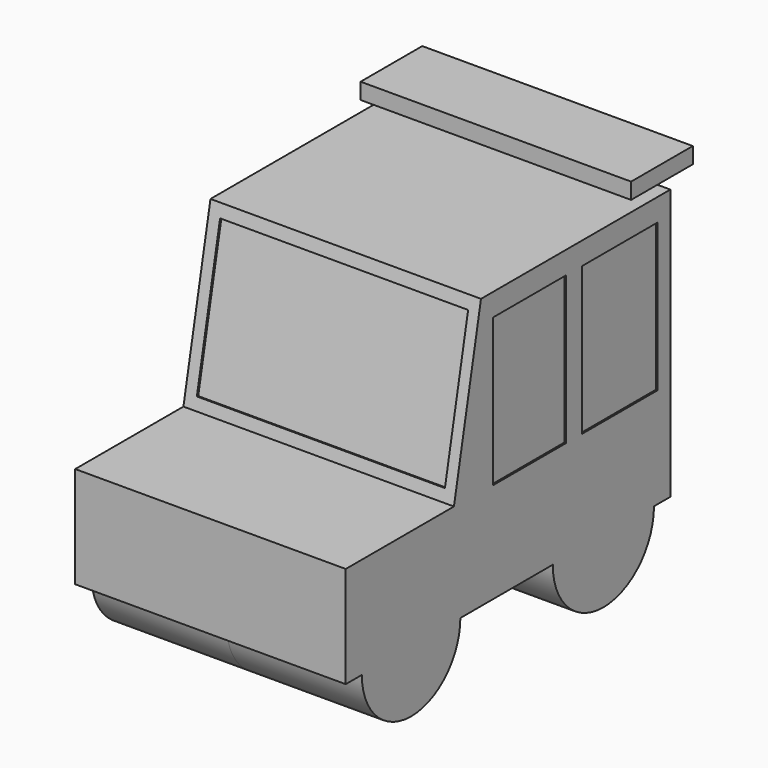
from build123d import *

# Parameters (mm, degrees)
F2_DEPTH  = 40
F1_R      = 18.2030638816
F1_R_2    = 18.7046022313
F3_DEPTH  = 40
F4_W      = 27.0581897348
F4_H      = 43.6939634383
F4_W_2    = 27.8599155135
F5_DEPTH  = 0.5
F6_W      = 73.3577571809
F6_H      = 43.7416750938
F7_DEPTH  = 0.5
F8_W      = 7.9477988183
F8_H      = 10.0772306323
F9_DEPTH  = 12.5
F10_W     = 22.8018909693
F10_H     = 4.7676712275
F11_DEPTH = 40


# Not quite as in the source:
# - a pattern or mirror of a feature is missing from the dataset's text; its kind, count and spacing are read off the source's solid
# - a feature names something its author has since deleted; it is built from what else it names


with BuildPart() as f2:
    # F0 (on Right) → F2 (new body, symmetric)
    with BuildSketch(Plane.YZ):
        Polygon((-85.6041714479, 30), (-85.6041714479, 0), (34.3958285521, 0), (34.3958285521, 80), (-35.6041714479, 80), (-45.6041714479, 30), align=None)
    extrude(amount=F2_DEPTH, both=True)

    # F1 (on Right) → F3 (join, symmetric)
    with BuildSketch(Plane.YZ):
        with Locations((-61.4385381341, 0)):
            Circle(F1_R)
        with Locations((9.633612819, 0)):
            Circle(F1_R_2)
    extrude(amount=F3_DEPTH, both=True)

    # F4 (on face) → F5 (cut, symmetric)
    with BuildSketch(Plane.YZ.offset(40)):
        with Locations((-17.7288064733, 51.5053849667)):
            Rectangle(F4_W, F4_H)
        with Locations((15.7431771513, 51.5053849667)):
            Rectangle(F4_W_2, F4_H)
    f5 = extrude(amount=F5_DEPTH, both=True, mode=Mode.SUBTRACT)

    # F5_copies: F5 across plane
    add(f5.mirror(Plane(origin=(0, 0, 0), x_dir=(0, 0, -1), z_dir=(-1, 0, 0))), mode=Mode.SUBTRACT)

    # F6 (on face) → F7 (cut, symmetric)
    with BuildSketch(Plane(origin=(0, -49.619395623, 9.9238791246), x_dir=(1, 0, 0), z_dir=(0, -0.9805806757, 0.1961161351))):
        with Locations((0.100215897, 45.8797877654)):
            Rectangle(F6_W, F6_H)
    extrude(amount=F7_DEPTH, both=True, mode=Mode.SUBTRACT)

    # F8 (on Right) → F9 (join, symmetric)
    with BuildSketch(Plane.YZ):
        with Locations((30.565129593, 80.2655704319)):
            Rectangle(F8_W, F8_H)
    extrude(amount=F9_DEPTH, both=True)

    # F10 (on Right) → F11 (join, symmetric)
    with BuildSketch(Plane.YZ):
        with Locations((31.2845855951, 85.5805724859)):
            Rectangle(F10_W, F10_H)
    extrude(amount=F11_DEPTH, both=True)


solid = f2.part
